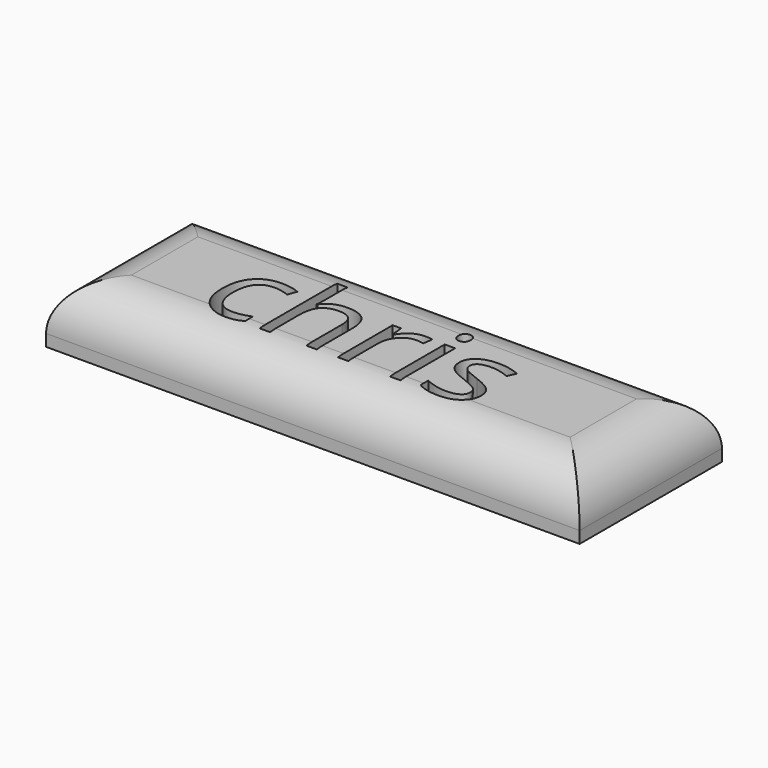
from build123d import *

# Parameters (mm, degrees)
F0_W         = 57.15
F0_H         = 19.05
F1_DEPTH     = 6.35
F2_TEXT_SIZE = 13.6612384166
F3_DEPTH     = 2.54
F4_T1_DEPTH  = 82.55
F4_T3_DEPTH  = 44.45


# Not quite as in the source:
# - a fillet or chamfer that OpenCascade refuses, or shapes differently, is made with other operations: its cross-section is extruded or revolved along the edge and cut away or added
# - Text() gives the source's letters only with a copy of the font that has no kerning and outlines rounded to 1/6400 em; it was checked with that copy


with BuildPart() as f1:
    # F0 (on Top) → F1 (new body)
    with BuildSketch(Plane.XY):
        with Locations((2.4468643785, -4.6470874235)):
            Rectangle(F0_W, F0_H)
    extrude(amount=F1_DEPTH)

    # F2 (on face) → F3 (cut)
    with BuildSketch(Plane.XY.offset(6.35)):
        with Locations((-14.3871179316, -9.83609166)):
            Text('chris', F2_TEXT_SIZE, font='Open Sans', text_align=(TextAlign.LEFT, TextAlign.BOTTOM))
    extrude(amount=-F3_DEPTH, mode=Mode.SUBTRACT)

    # F4: fillet of radius 5.08 on 4 edges, made by hand

    # F4_s2 → F4_t1 (cut)
    with BuildSketch(Plane.YZ.offset(-38.8281356215)):
        with BuildLine():
            ThreePointArc((4.8779125765, 1.27), (3.3900150249, 4.8621024484), (-0.2020874235, 6.35))
            Line((-0.2020874235, 6.35), (4.8779125765, 6.35))
            Line((4.8779125765, 6.35), (4.8779125765, 1.27))
        make_face()
        with BuildLine():
            ThreePointArc((-9.0920874235, 6.35), (-12.6841898719, 4.8621024484), (-14.1720874235, 1.27))
            Line((-14.1720874235, 1.27), (-14.1720874235, 6.35))
            Line((-14.1720874235, 6.35), (-9.0920874235, 6.35))
        make_face()
    extrude(amount=F4_T1_DEPTH, mode=Mode.SUBTRACT)

    # F4_s4 → F4_t3 (cut)
    with BuildSketch(Plane.XZ.offset(-17.5779125765)):
        with BuildLine():
            ThreePointArc((-26.1281356215, 1.27), (-24.64023807, 4.8621024484), (-21.0481356215, 6.35))
            Line((-21.0481356215, 6.35), (-26.1281356215, 6.35))
            Line((-26.1281356215, 6.35), (-26.1281356215, 1.27))
        make_face()
        with BuildLine():
            ThreePointArc((31.0218643785, 1.27), (29.5339668269, 4.8621024484), (25.9418643785, 6.35))
            Line((25.9418643785, 6.35), (31.0218643785, 6.35))
            Line((31.0218643785, 6.35), (31.0218643785, 1.27))
        make_face()
    extrude(amount=F4_T3_DEPTH, mode=Mode.SUBTRACT)


solid = f1.part
